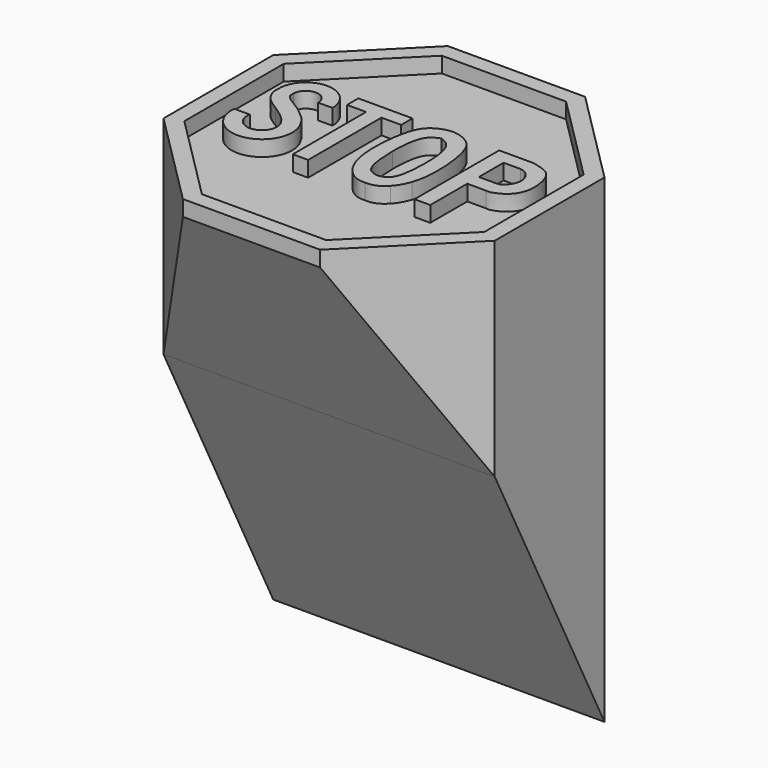
from build123d import *

# Parameters (mm, degrees)
F1_DEPTH   = 88.9
F1_FACE1_W = 26.3025612107
F1_FACE1_H = 88.9
F3_DEPTH   = 63.5
F5_DEPTH   = 3


# Not quite as in the source:
# - a feature names something its author has since deleted; it is built from what else it names


with BuildPart() as f1:
    # F0 (on Top) → F1 (new body)
    with BuildSketch(Plane.XY):
        Polygon((13.1512806053, 31.75), (-13.1512806053, 31.75), (-31.75, 13.1512806053), (-31.75, -13.1512806053), (-13.1512806053, -31.75), (13.1512806053, -31.75), (31.75, -13.1512806053), (31.75, 13.1512806053), align=None)
    extrude(amount=-F1_DEPTH)

    # F2 (on face) + F1_face1 (on face) → F3 (cut, through all)
    with BuildSketch(Plane(origin=(-31.75, 0, 0), x_dir=(0, -1, 0), z_dir=(-1, 0, 0))):
        Polygon((-19.05, -88.9), (-31.75, 0), (-31.75, -88.9), align=None)
        Polygon((31.75, -88.9), (31.75, 0), (13.1512806053, -36.823585695), (13.1512806053, -88.9), (14.6601814777, -88.9), align=None)
        Polygon((13.1512806053, -36.823585695), (-13.1512806053, -88.9), (-12.7, -88.9), (-6.35, -88.9), (0, -88.9), (8.3101814777, -88.9), (13.1512806053, -88.9), align=None)
    with BuildSketch(Plane(origin=(22.4506403027, -22.4506403027, -44.45), x_dir=(0.7071067812, 0.7071067812, 0), z_dir=(0.7071067812, -0.7071067812, 0))):
        Rectangle(F1_FACE1_W, F1_FACE1_H)
    extrude(amount=-F3_DEPTH, dir=(-1, 0, 0), mode=Mode.SUBTRACT)

    # F4 (on face) → F5 (join)
    with BuildSketch(Plane.XY):
        Polygon((13.1512806053, 31.75), (-13.1512806053, 31.75), (-31.75, 13.1512806053), (-31.75, -13.1512806053), (-13.1512806053, -31.75), (13.1512806053, -31.75), (31.75, -13.1512806053), (31.75, 13.1512806053), align=None)
        Polygon((-28.75, 10.7754608616), (-28.75, 11.9086399182), (-11.9086399182, 28.75), (11.9086399182, 28.75), (28.75, 11.9086399182), (28.75, 10.7754608616), (28.75, -10.7754608616), (28.75, -11.9086399182), (11.9086399182, -28.75), (-11.9086399182, -28.75), (-28.75, -11.9086399182), (-28.75, -10.7754608616), align=None, mode=Mode.SUBTRACT)
        with BuildLine():
            add(Edge.make_bspline(
                [(4.8083327711, 10.5354869738), (5.9249649259, 10.4834162819), (7.339599469, 10.0059956165), (8.3643975774, 9.1943899894), (8.5739761095, 8.9890481737)],
                knots=[0, 0, 0, 0, 0.0796423572, 0.1022272486, 0.1022272486, 0.1022272486, 0.1022272486], degree=3))
            add(Edge.make_bspline(
                [(4.8083327711, 10.5354869738), (3.6917006162, 10.4834162819), (2.2770660731, 10.0059956165), (1.2522679647, 9.1943899894), (1.0426894326, 8.9890481737)],
                knots=[0, 0, 0, 0, 0.0796423572, 0.1022272486, 0.1022272486, 0.1022272486, 0.1022272486], degree=3))
            add(Edge.make_bspline(
                [(-0.5542273499, -6.0097523046), (-0.6853048791, -5.4911473404), (-1.2029837025, -2.5307480598), (-1.3645767848, 4.0861219904), (0.1727738224, 7.9642019091), (1.0426894326, 8.9890481737)],
                knots=[0.6521796741, 0.6521796741, 0.6521796741, 0.6521796741, 0.683293281, 0.8153772216, 0.9015400151, 0.9015400151, 0.9015400151, 0.9015400151], degree=3))
            add(Edge.make_bspline(
                [(-0.5542273499, -6.0097523046), (-0.1219359708, -7.2774050993), (0.4855176774, -8.258165167), (1.158925978, -8.9826247772)],
                knots=[0.3319618275, 0.3319618275, 0.3319618275, 0.3319618275, 0.3946519049, 0.3946519049, 0.3946519049, 0.3946519049], degree=3))
            add(Edge.make_bspline(
                [(4.8083327711, -10.5354869738), (3.6099604652, -10.4237469099), (2.1738291685, -9.8473995471), (1.158925978, -8.9826247772)],
                knots=[0.4948947439, 0.4948947439, 0.4948947439, 0.4948947439, 0.5783031472, 0.5783031472, 0.5783031472, 0.5783031472], degree=3))
            add(Edge.make_bspline(
                [(4.8083327711, -10.5354869738), (6.0067050769, -10.4237469099), (7.4428363737, -9.8473995471), (8.4577395641, -8.9826247772)],
                knots=[0.4948947439, 0.4948947439, 0.4948947439, 0.4948947439, 0.5783031472, 0.5783031472, 0.5783031472, 0.5783031472], degree=3))
            add(Edge.make_bspline(
                [(10.170892892, -6.0097523046), (9.7386015129, -7.2774050993), (9.1311478647, -8.258165167), (8.4577395641, -8.9826247772)],
                knots=[0.3319618275, 0.3319618275, 0.3319618275, 0.3319618275, 0.3946519049, 0.3946519049, 0.3946519049, 0.3946519049], degree=3))
            add(Edge.make_bspline(
                [(10.170892892, -6.0097523046), (10.3019704212, -5.4911473404), (10.8196492446, -2.5307480598), (10.9812423269, 4.0861219904), (9.4438917197, 7.9642019091), (8.5739761095, 8.9890481737)],
                knots=[0.6521796741, 0.6521796741, 0.6521796741, 0.6521796741, 0.683293281, 0.8153772216, 0.9015400151, 0.9015400151, 0.9015400151, 0.9015400151], degree=3))
        make_face()
        with BuildLine():
            add(Edge.make_bspline(
                [(4.8083327711, 7.7876993455), (3.9534414496, 7.4218723248), (2.0820207972, 6.6210497822), (1.660966503, 2.272494011), (1.6738338819, 0)],
                knots=[0, 0, 0, 0, 0.2110894815, 0.4620905666, 0.4620905666, 0.4620905666, 0.4620905666], degree=3))
            add(Edge.make_bspline(
                [(4.8083327711, 7.7876993455), (5.6632240926, 7.4218723248), (8.028214212, 6.4098404237), (8.0974839635, -3.0892679636), (6.9910117402, -7.135194286), (5.4397234852, -7.47767614), (4.8083327711, -7.617069874)],
                knots=[0, 0, 0, 0, 0.2110894815, 0.5839625756, 0.8306683715, 1, 1, 1, 1], degree=3))
            add(Edge.make_bspline(
                [(1.6738338819, 0), (1.6800815574, -1.1033952726), (1.8712186248, -4.3765266238), (2.6256538019, -7.135194286), (4.1769420569, -7.47767614), (4.8083327711, -7.617069874)],
                knots=[0.4620905666, 0.4620905666, 0.4620905666, 0.4620905666, 0.5839625756, 0.8306683715, 1, 1, 1, 1], degree=3))
        make_face(mode=Mode.SUBTRACT)
        with BuildLine():
            Line((20.6052474678, 10.1401684806), (13.9625072479, 10.1401684806))
            Line((13.9625072479, 10.1401684806), (13.9625072479, -10.1387687027))
            Line((13.9625072479, -10.1387687027), (16.9827528298, -10.1387687027))
            Line((16.9827528298, -10.1387687027), (16.9827528298, -1.2698972132))
            Line((16.9827528298, -1.2698972132), (20.6052474678, -1.2698972132))
            add(Edge.make_bspline(
                [(20.6052474678, 10.1401684806), (21.8779731079, 9.8412745125), (24.3142685907, 9.2691213309), (25.4822457744, 6.1351724103), (25.736421693, 2.6562033682), (24.2123159942, -0.1800935194), (21.4538469207, -1.3948664952), (20.8225355964, -1.3018962221), (20.6052474678, -1.2698972132)],
                knots=[0, 0, 0, 0, 0.1937641782, 0.3709100981, 0.5596905933, 0.7399766879, 0.9105037773, 1, 1, 1, 1], degree=3))
        make_face()
        with BuildLine():
            Line((20.2160011977, 1.5110635431), (16.9827528298, 1.5110635431))
            Line((16.9827528298, 1.5110635431), (16.9827528298, 7.4263564311))
            Line((16.9827528298, 7.4263564311), (20.2160011977, 7.4263564311))
            add(Edge.make_bspline(
                [(20.2160011977, 7.4263564311), (21.1544893682, 7.4114310555), (22.7486394765, 6.0097179724), (22.8736105917, 3.1708769977), (21.149745211, 1.4233636903), (20.2160011977, 1.5110635431)],
                knots=[0, 0, 0, 0, 0.3295814167, 0.6602854532, 1, 1, 1, 1], degree=3))
        make_face(mode=Mode.SUBTRACT)
        with BuildLine():
            ThreePointArc((-16.8338958174, -4.1077076457), (-19.6410734206, -7.564034438), (-22.4482510239, -4.1077076457))
            Line((-22.4482510239, -4.1077076457), (-25.4293251783, -4.1077076457))
            ThreePointArc((-25.4293251783, -4.1077076457), (-18.1588622297, -10.3219857216), (-14.8939756829, -1.3321359272))
            add(Edge.make_bspline(
                [(-15.8727969974, 0), (-15.4709741473, -0.3938739537), (-15.0835029781, -0.853099511), (-14.8939756829, -1.3321359272)],
                knots=[0, 0, 0, 0, 1.6530811518, 1.6530811518, 1.6530811518, 1.6530811518], degree=3))
            add(Edge.make_bspline(
                [(-21.5829703957, 5.279887002), (-21.6180322262, 4.9093177243), (-21.7144690872, 3.8900743649), (-18.3106174987, 2.2689761454), (-16.6874966749, 0.7582732743), (-15.8727969974, 0)],
                knots=[0, 0, 0, 0, 0.221505784, 0.6092472123, 1, 1, 1, 1], degree=3))
            ThreePointArc((-21.5829703957, 5.279887002), (-19.2209649831, 7.6604824432), (-16.8589595705, 5.279887002))
            Line((-16.8589595705, 5.279887002), (-14.1183091328, 5.3153838962))
            ThreePointArc((-14.1183091328, 5.3153838962), (-19.22945472, 10.4010814839), (-24.3236490835, 5.298404446))
            add(Edge.make_bspline(
                [(-24.3236490835, 5.298404446), (-24.3557528234, 4.7439102233), (-24.4260352796, 3.5299950823), (-23.0471913533, 1.3752329572), (-21.5360686477, 0.4670374949), (-20.7589771599, 0)],
                knots=[0, 0, 0, 0, 0.2900044831, 0.6348863858, 1, 1, 1, 1], degree=3))
            add(Edge.make_bspline(
                [(-20.7589771599, 0), (-19.6156120227, -0.7838167648), (-18.2336909625, -1.7311719529), (-17.5404152252, -2.6957135463), (-17.4353591755, -2.8625837034)],
                knots=[0, 0, 0, 0, 0.5794694701, 0.7003721194, 0.7003721194, 0.7003721194, 0.7003721194], degree=3))
            ThreePointArc((-17.4353591755, -2.8625837034), (-17.0584672604, -3.448356091), (-16.8338958174, -4.1077076457))
        make_face()
        Polygon((-9.3714222312, 7.4263564311), (-9.3714222312, -10.1387687027), (-6.427643355, -10.1387687027), (-6.427643355, 7.4263564311), (-2.6484197006, 7.4263564311), (-2.6484197006, 10.1401684806), (-6.427643355, 10.1401684806), (-9.3714222312, 10.1401684806), (-13.0321141332, 10.1401684806), (-13.0321141332, 7.4263564311), align=None)
        with BuildLine():
            add(Edge.make_bspline(
                [(-0.5542273499, -6.0097523046), (-0.6853048791, -5.4911473404), (-1.2029837025, -2.5307480598), (-1.3645767848, 4.0861219904), (0.1727738224, 7.9642019091), (1.0426894326, 8.9890481737)],
                knots=[0.6521796741, 0.6521796741, 0.6521796741, 0.6521796741, 0.683293281, 0.8153772216, 0.9015400151, 0.9015400151, 0.9015400151, 0.9015400151], degree=3))
            add(Edge.make_bspline(
                [(1.0426894326, 8.9890481737), (0.4633846395, 8.4214542659), (-1.0609269861, 5.8291860693), (-1.6974790085, -2.0230291515), (-0.6825603591, -5.6334281267), (-0.5542273499, -6.0097523046)],
                knots=[0.1022272486, 0.1022272486, 0.1022272486, 0.1022272486, 0.1646550922, 0.3133512175, 0.3319618275, 0.3319618275, 0.3319618275, 0.3319618275], degree=3))
        make_face()
        with BuildLine():
            add(Edge.make_bspline(
                [(8.5739761095, 8.9890481737), (9.1532809026, 8.4214542659), (10.6775925282, 5.8291860693), (11.3141445506, -2.0230291515), (10.2992259012, -5.6334281267), (10.170892892, -6.0097523046)],
                knots=[0.1022272486, 0.1022272486, 0.1022272486, 0.1022272486, 0.1646550922, 0.3133512175, 0.3319618275, 0.3319618275, 0.3319618275, 0.3319618275], degree=3))
            add(Edge.make_bspline(
                [(10.170892892, -6.0097523046), (10.3019704212, -5.4911473404), (10.8196492446, -2.5307480598), (10.9812423269, 4.0861219904), (9.4438917197, 7.9642019091), (8.5739761095, 8.9890481737)],
                knots=[0.6521796741, 0.6521796741, 0.6521796741, 0.6521796741, 0.683293281, 0.8153772216, 0.9015400151, 0.9015400151, 0.9015400151, 0.9015400151], degree=3))
        make_face()
        with BuildLine():
            add(Edge.make_bspline(
                [(4.8083327711, -10.5354869738), (3.6099604652, -10.4237469099), (2.1738291685, -9.8473995471), (1.158925978, -8.9826247772)],
                knots=[0.4948947439, 0.4948947439, 0.4948947439, 0.4948947439, 0.5783031472, 0.5783031472, 0.5783031472, 0.5783031472], degree=3))
            add(Edge.make_bspline(
                [(1.158925978, -8.9826247772), (1.4164965069, -9.2597218145), (2.5336297837, -10.2613938856), (3.712598623, -10.6376567279), (4.8083327711, -10.5354869738)],
                knots=[0.3946519049, 0.3946519049, 0.3946519049, 0.3946519049, 0.4186301011, 0.4948947439, 0.4948947439, 0.4948947439, 0.4948947439], degree=3))
        make_face()
        with BuildLine():
            add(Edge.make_bspline(
                [(8.4577395641, -8.9826247772), (8.2001690352, -9.2597218145), (7.0830357584, -10.2613938856), (5.9040669191, -10.6376567279), (4.8083327711, -10.5354869738)],
                knots=[0.3946519049, 0.3946519049, 0.3946519049, 0.3946519049, 0.4186301011, 0.4948947439, 0.4948947439, 0.4948947439, 0.4948947439], degree=3))
            add(Edge.make_bspline(
                [(4.8083327711, -10.5354869738), (6.0067050769, -10.4237469099), (7.4428363737, -9.8473995471), (8.4577395641, -8.9826247772)],
                knots=[0.4948947439, 0.4948947439, 0.4948947439, 0.4948947439, 0.5783031472, 0.5783031472, 0.5783031472, 0.5783031472], degree=3))
        make_face()
    extrude(amount=F5_DEPTH)


solid = f1.part
